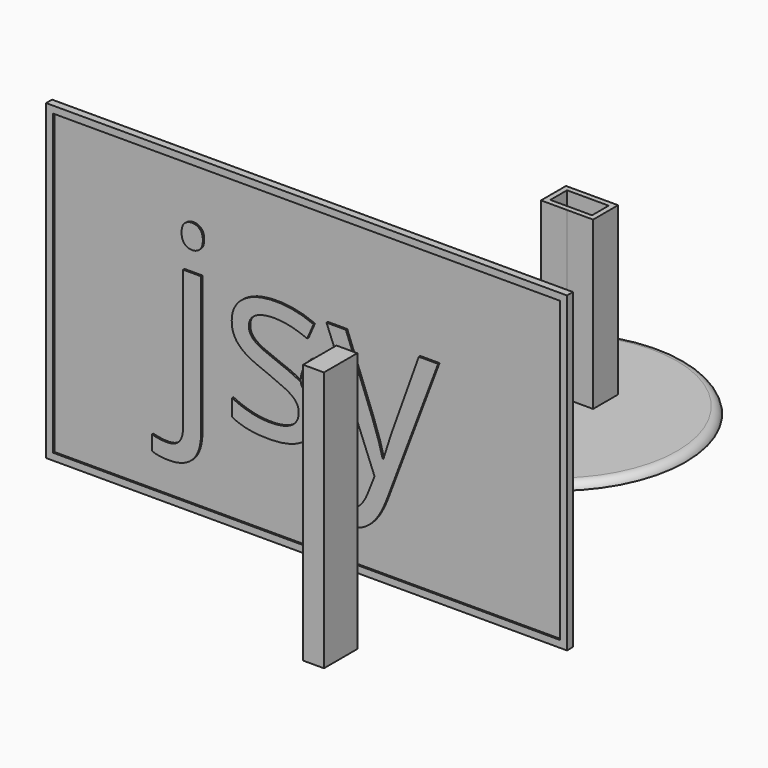
from build123d import *

# Parameters (mm, degrees)
F0_W          = 300
F0_H          = 180
F0_W_2        = 292
F0_H_2        = 172
F1_DEPTH      = 5
F2_DEPTH      = 4
F3_R          = 1
F4_R          = 75
F5_DEPTH      = 4
F6_DEPTH      = 100
F9_DEPTH      = 15
F10_R         = 5
F11_W         = 24
F11_H         = 150
F11_R         = 7.5
F12_DEPTH     = 12
F13_DEPTH     = 5
F14_R         = 7.5
F15_DEPTH     = 3
F16_TEXT_SIZE = 128.0613722176
F17_DEPTH     = 1


# Not quite as in the source:
# - a fillet or chamfer that OpenCascade refuses, or shapes differently, is made with other operations: its cross-section is extruded or revolved along the edge and cut away or added
# - a feature names something its author has since deleted; it is built from what else it names
# - Text() gives the source's letters only with a copy of the font that has no kerning and outlines rounded to 1/6400 em; it was checked with that copy


with BuildPart() as f1:
    # F0 (on Front) → F1 (new body)
    with BuildSketch(Plane.XZ):
        with Locations((-30, 66.6834676266)):
            Rectangle(F0_W, F0_H)
        with Locations((-30, 66.6834676266)):
            Rectangle(F0_W_2, F0_H_2, mode=Mode.SUBTRACT)
    extrude(amount=F1_DEPTH)

    # F0 (on Front) → F2 (join)
    with BuildSketch(Plane.XZ):
        with Locations((-30, 66.6834676266)):
            Rectangle(F0_W_2, F0_H_2)
        Polygon((0, 47.6834676266), (0, 36.6834676266), (-60, 36.6834676266), (-60, 47.6834676266), (-60, 74.6559426188), (0, 74.6559426188), align=None, mode=Mode.SUBTRACT)
        Polygon((-60, 36.6834676266), (0, 36.6834676266), (0, 47.6834676266), (0, 74.6559426188), (-60, 74.6559426188), (-60, 47.6834676266), align=None)
    extrude(amount=F2_DEPTH)

    # F3
    f3_edges = [f1.edges().sort_by_distance(p)[0] for p in [
        (-30, 0, -23.316532),
        (-180, 0, 66.683468),
        (-30, 0, 156.683468),
        (120, 0, 66.683468),
    ]]
    fillet(f3_edges, radius=F3_R)

    # F0 (on Front) → F9 (join)
    with BuildSketch(Plane.XZ):
        Polygon((-60, 36.6834676266), (0, 36.6834676266), (0, 47.6834676266), (0, 74.6559426188), (-60, 74.6559426188), (-60, 47.6834676266), align=None)
    extrude(amount=-F9_DEPTH)

    # F10
    f10_edges = [f1.edges().sort_by_distance(p)[0] for p in [
        (-30, 15, 36.683468),
        (0, 15, 55.669705),
        (-30, 15, 74.655943),
        (-60, 15, 55.669705),
    ]]
    fillet(f10_edges, radius=F10_R)

    # F14 (on face) → F15 (cut)
    with BuildSketch(Plane(origin=(0, 15, 0), x_dir=(-1, 0, 0), z_dir=(0, 1, 0))):
        with Locations((30, 55.6697051227)):
            Circle(F14_R)
    extrude(amount=-F15_DEPTH, mode=Mode.SUBTRACT)

    # F16 (on offset) → F17 (join, through all)
    with BuildSketch(Plane.XZ.offset(5)):
        with Locations((-112.1006067842, 29.3302936479)):
            Text('jsy', F16_TEXT_SIZE, font='Open Sans', text_align=(TextAlign.LEFT, TextAlign.BOTTOM))
    extrude(amount=-F17_DEPTH)


with BuildPart() as f5:
    # F4 (on Top) → F5 (new body)
    with BuildSketch(Plane.XY):
        with Locations((0, 136.687554419)):
            Circle(F4_R)
        Polygon((0, 145.0392252011), (-15, 145.0352982098), (-15, 163.0352982098), (15, 163.0352982098), (15, 145.0431521923), align=None, mode=Mode.SUBTRACT)
        Polygon((-15, 163.0352982098), (-15, 145.0352982098), (0, 145.0392252011), (15, 145.0431521923), (15, 163.0352982098), align=None)
        Polygon((-12, 148.0360837109), (-12, 160.0352982098), (0, 160.0352982098), (12, 160.0352982098), (12, 148.0423668969), align=None, mode=Mode.SUBTRACT)
        Polygon((0, 160.0352982098), (-12, 160.0352982098), (-12, 148.0360837109), (12, 148.0423668969), (12, 160.0352982098), align=None)
    extrude(amount=F5_DEPTH)

    # F4 (on Top) → F6 (join)
    with BuildSketch(Plane.XY):
        Polygon((-15, 163.0352982098), (-15, 145.0352982098), (0, 145.0392252011), (15, 145.0431521923), (15, 163.0352982098), align=None)
        Polygon((-12, 148.0360837109), (-12, 160.0352982098), (0, 160.0352982098), (12, 160.0352982098), (12, 148.0423668969), align=None, mode=Mode.SUBTRACT)
    extrude(amount=F6_DEPTH)

    # F7: fillet of radius 5 on 1 edges, made by hand

    # F7_s1 → F7_t2 (revolve, cut)
    with BuildSketch(Plane.XZ.offset(-136.687554419)):
        with BuildLine():
            ThreePointArc((75, 0), (73.2632981746, 2.8729833462), (70.1010205144, 4))
            Line((70.1010205144, 4), (75, 4))
            Line((75, 4), (75, 0))
        make_face()
    revolve(axis=Axis((0, 136.687554419, 4), (0, 0, 1)), mode=Mode.SUBTRACT)


with BuildPart() as f12:
    # F11 (on Right) → F12 (new body)
    with BuildSketch(Plane.YZ):
        with Locations((-32.9572475664, 23.7755745649)):
            Rectangle(F11_W, F11_H)
        with Locations((-32.9572475664, 87.4674811286)):
            Circle(F11_R, mode=Mode.SUBTRACT)
        with Locations((-32.9572475664, 87.4674811286)):
            Circle(F11_R)
    extrude(amount=F12_DEPTH)

    # F11 (on Right) → F13 (join)
    with BuildSketch(Plane.YZ):
        with Locations((-32.9572475664, 87.4674811286)):
            Circle(F11_R)
    extrude(amount=-F13_DEPTH)


solid = Compound([f1.part, f5.part, f12.part])
